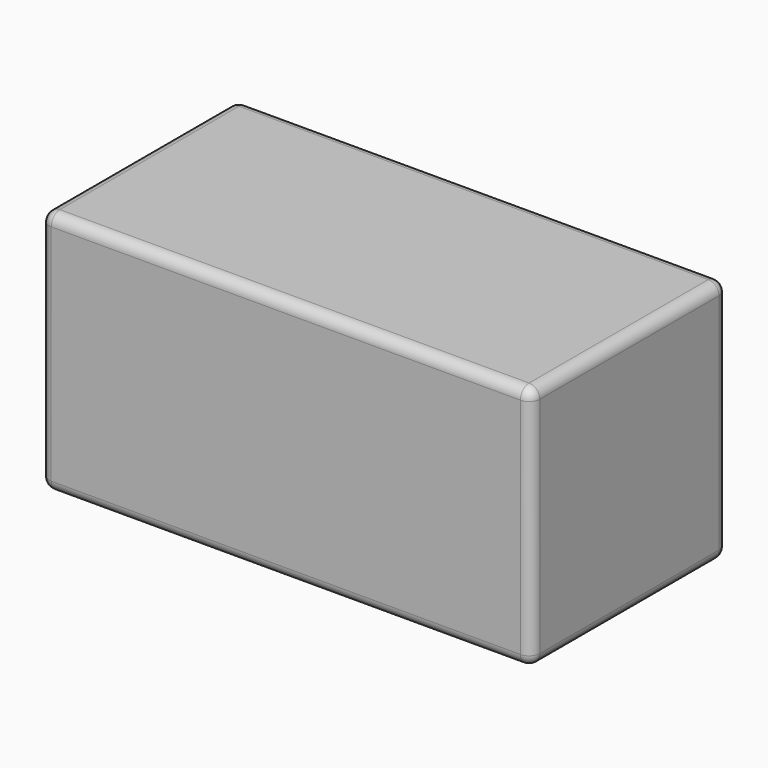
from build123d import *

# Parameters (mm, degrees)
F1_DEPTH             = 34.2
F2_W                 = 34.2
F2_H                 = 34.2
F3_DEPTH             = 34.2
F4_W                 = 28.2
F4_H                 = 28.2
F5_DEPTH             = 31.2
F8_D                 = 3.3
F8_DEPTH             = 25
F8_CSINK_D           = 6.72
F8_CSINK_ANGLE       = 90
F8_TIP               = 0.9914200214
F8_ON_F7_D           = 3.3
F8_ON_F7_DEPTH       = 25
F8_ON_F7_CSINK_D     = 6.72
F8_ON_F7_CSINK_ANGLE = 90
F8_ON_F7_TIP         = 0.9914200214
F9_W                 = 28.2
F9_H                 = 28.2
F10_DEPTH            = 31.2
F11_R                = 1.49999
F12_W                = 5
F12_H                = 5
F13_DEPTH            = 2.5


# Not quite as in the source:
# - a fillet or chamfer is up to 0.001 mm smaller than in the source, because OpenCascade refuses the exact size
# - a feature names something its author has since deleted; it is built from what else it names


with BuildPart() as f1:
    # F0 (on Top) → F1 (new body)
    with BuildSketch(Plane.XY):
        Polygon((-34.2, 0), (-8, 0), (0, 0), (0, 34.2), (-34.2, 34.2), align=None)
    extrude(amount=F1_DEPTH)

    # F2 (on face) → F3 (join)
    with BuildSketch(Plane(origin=(-34.2, 0, 0), x_dir=(0, -1, 0), z_dir=(-1, 0, 0))):
        with Locations((-17.1, 17.1)):
            Rectangle(F2_W, F2_H)
    extrude(amount=F3_DEPTH)

    # F4 (on face) → F5 (cut)
    with BuildSketch(Plane(origin=(-68.4, 0, 0), x_dir=(0, -1, 0), z_dir=(-1, 0, 0))):
        with Locations((-17.1, 17.1)):
            Rectangle(F4_W, F4_H)
    extrude(amount=-F5_DEPTH, mode=Mode.SUBTRACT)

    # F8
    with Locations(Plane(origin=(0, 34.2, 0), x_dir=(-1, 0, 0), z_dir=(0, 1, 0))):
        with Locations((17.05, 17.1), (51.35, 17.1)):
            CounterSinkHole(F8_D / 2, F8_CSINK_D / 2, depth=F8_DEPTH, counter_sink_angle=F8_CSINK_ANGLE)
            with Locations((0, 0, -(F8_DEPTH + F8_TIP / 2))):  # 118° drill point
                Cone(0, F8_D / 2, F8_TIP, mode=Mode.SUBTRACT)

    # F8 on F7
    with Locations(Plane(origin=(-37.2, 0, 0), x_dir=(0, -1, 0), z_dir=(-1, 0, 0))):
        with Locations((-17.1, 17.1)):
            CounterSinkHole(F8_ON_F7_D / 2, F8_ON_F7_CSINK_D / 2, depth=F8_ON_F7_DEPTH, counter_sink_angle=F8_ON_F7_CSINK_ANGLE)
            with Locations((0, 0, -(F8_ON_F7_DEPTH + F8_ON_F7_TIP / 2))):  # 118° drill point
                Cone(0, F8_ON_F7_D / 2, F8_ON_F7_TIP, mode=Mode.SUBTRACT)

    # F9 (on face) → F10 (cut)
    with BuildSketch(Plane(origin=(0, 0, 0), x_dir=(1, 0, 0), z_dir=(0, 0, -1))):
        with Locations((-17.1, -17.1)):
            Rectangle(F9_W, F9_H)
    extrude(amount=-F10_DEPTH, mode=Mode.SUBTRACT)

    # F11 (radius 1.5 in the source; OpenCascade refuses exactly that, so slightly less here)
    f11_edges = [f1.edges().sort_by_distance(p)[0] for p in [
        (-31.2, 17.1, 0),
        (-17.1, 3, 0),
        (-3, 17.1, 0),
        (-17.1, 31.2, 0),
        (-34.2, 34.2, 0),
        (-34.2, 0, 0),
        (0, 17.1, 0),
        (-68.4, 17.1, 0),
        (-68.4, 0, 17.1),
        (-68.4, 17.1, 34.2),
        (-68.4, 34.2, 17.1),
        (-68.4, 17.1, 31.2),
        (-68.4, 3, 17.1),
        (-68.4, 17.1, 3),
        (-68.4, 31.2, 17.1),
        (-34.2, 0, 34.2),
        (-34.2, 34.2, 34.2),
        (0, 17.1, 34.2),
        (0, 34.2, 17.1),
        (0, 0, 17.1),
    ]]
    fillet(f11_edges, radius=F11_R)

    # F12 (on face) → F13 (cut)
    with BuildSketch(Plane(origin=(0, 34.2, 0), x_dir=(-1, 0, 0), z_dir=(0, 1, 0))):
        with Locations((14.5, 25.7)):
            Rectangle(F12_W, F12_H)
    extrude(amount=-F13_DEPTH, mode=Mode.SUBTRACT)


solid = f1.part
